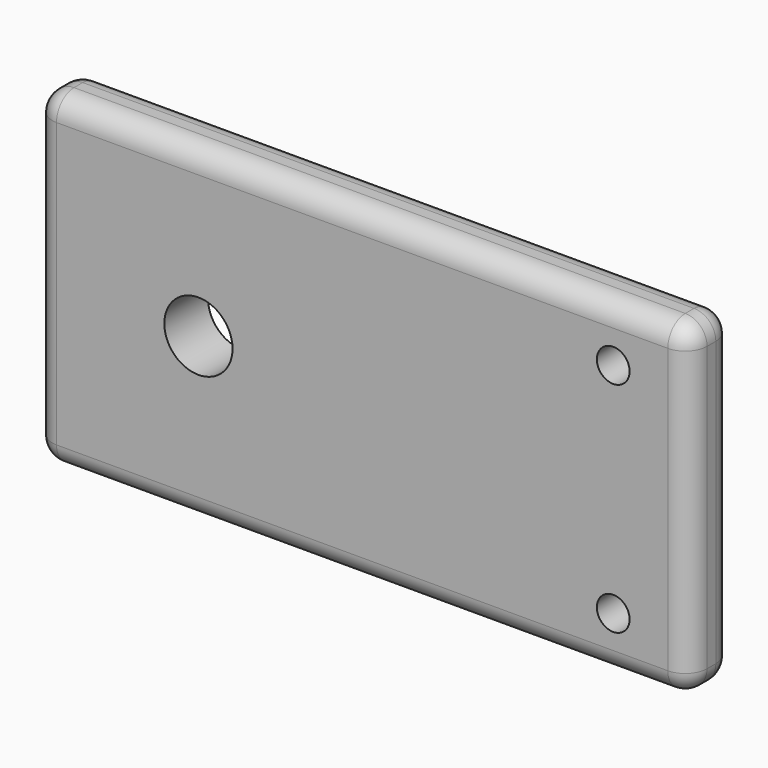
from build123d import *

# Parameters (mm, degrees)
F0_W         = 152.4
F0_H         = 76.2
F0_R         = 7.9375
F1_DEPTH     = 6.35
F2_R         = 5.08
F3_T1_DEPTH  = 2.54
F3_S5_W      = 5.08
F3_S5_H      = 5.08
F3_T6_DEPTH  = 5.08
F3_S11_W     = 5.08
F3_S11_H     = 5.08
F3_T12_DEPTH = 5.08
F4_R         = 3.81
F5_DEPTH     = 25.4


# Not quite as in the source:
# - a fillet or chamfer that OpenCascade refuses, or shapes differently, is made with other operations: its cross-section is extruded or revolved along the edge and cut away or added


with BuildPart() as f1:
    # F0 (on Front) → F1 (new body, symmetric)
    with BuildSketch(Plane.XZ):
        Rectangle(F0_W, F0_H)
        with Locations((-38.1, 0)):
            Circle(F0_R, mode=Mode.SUBTRACT)
    extrude(amount=F1_DEPTH, both=True)

    # F2
    f2_edges = [f1.edges().sort_by_distance(p)[0] for p in [
        (0, -6.35, 38.1),
        (-76.2, -6.35, 0),
        (0, -6.35, -38.1),
        (76.2, -6.35, 0),
        (-76.2, 6.35, 0),
        (-76.2, 0, -38.1),
        (0, 6.35, -38.1),
        (76.2, 6.35, 0),
        (76.2, 0, -38.1),
        (76.2, 0, 38.1),
        (0, 6.35, 38.1),
    ]]
    fillet(f2_edges, radius=F2_R)

    # F3: fillet of radius 5.08 on 1 edges, made by hand

    # F3_s2 → F3_t1 (cut)
    with BuildSketch(Plane.XZ.offset(-1.27)):
        with BuildLine():
            ThreePointArc((-76.2, 33.02), (-74.7121024484, 36.6121024484), (-71.12, 38.1))
            Line((-71.12, 38.1), (-76.2, 38.1))
            Line((-76.2, 38.1), (-76.2, 33.02))
        make_face()
    extrude(amount=F3_T1_DEPTH, mode=Mode.SUBTRACT)


with BuildPart() as f3_tool4:
    # F3_s5 → F3_t6 (new body)
    with BuildSketch(Plane.YZ.offset(-71.12)):
        with Locations((-3.81, 35.56)):
            Rectangle(F3_S5_W, F3_S5_H)
    extrude(amount=-F3_T6_DEPTH)

    # F3_s7 → F3_t8 (revolve, cut)
    with BuildSketch(Plane(origin=(-71.12, -1.27, 33.02), x_dir=(0, 0.7071067812, -0.7071067812), z_dir=(0, 0.7071067812, 0.7071067812))):
        with BuildLine():
            ThreePointArc((0, -5.08), (5.08, 0), (0, 5.08))
            Line((0, 5.08), (0, -5.08))
        make_face()
    revolve(axis=Axis((-71.12, -1.27, 33.02), (-1, 0, 0)), mode=Mode.SUBTRACT)


with BuildPart() as f1_1:
    add(f1.part)

    # F3_t3: cut F3_tool4
    add(f3_tool4.part, mode=Mode.SUBTRACT)


with BuildPart() as f3_tool10:
    # F3_s11 → F3_t12 (new body)
    with BuildSketch(Plane.YZ.offset(-71.12)):
        with Locations((3.81, 35.56)):
            Rectangle(F3_S11_W, F3_S11_H)
    extrude(amount=-F3_T12_DEPTH)

    # F3_s13 → F3_t14 (revolve, cut)
    with BuildSketch(Plane(origin=(-71.12, 1.27, 33.02), x_dir=(0, -0.7071067812, -0.7071067812), z_dir=(0, 0.7071067812, -0.7071067812))):
        with BuildLine():
            ThreePointArc((0, -5.08), (5.08, 0), (0, 5.08))
            Line((0, 5.08), (0, -5.08))
        make_face()
    revolve(axis=Axis((-71.12, 1.27, 33.02), (-1, 0, 0)), mode=Mode.SUBTRACT)


with BuildPart() as f1_2:
    add(f1_1.part)

    # F3_t9: cut F3_tool10
    add(f3_tool10.part, mode=Mode.SUBTRACT)

    # F4 (on face) → F5 (cut)
    with BuildSketch(Plane.XZ.offset(6.35)):
        with Locations((58.42, 25.4)):
            Circle(F4_R)
        with Locations((58.42, -25.4)):
            Circle(F4_R)
    extrude(amount=-F5_DEPTH, mode=Mode.SUBTRACT)


solid = f1_2.part
